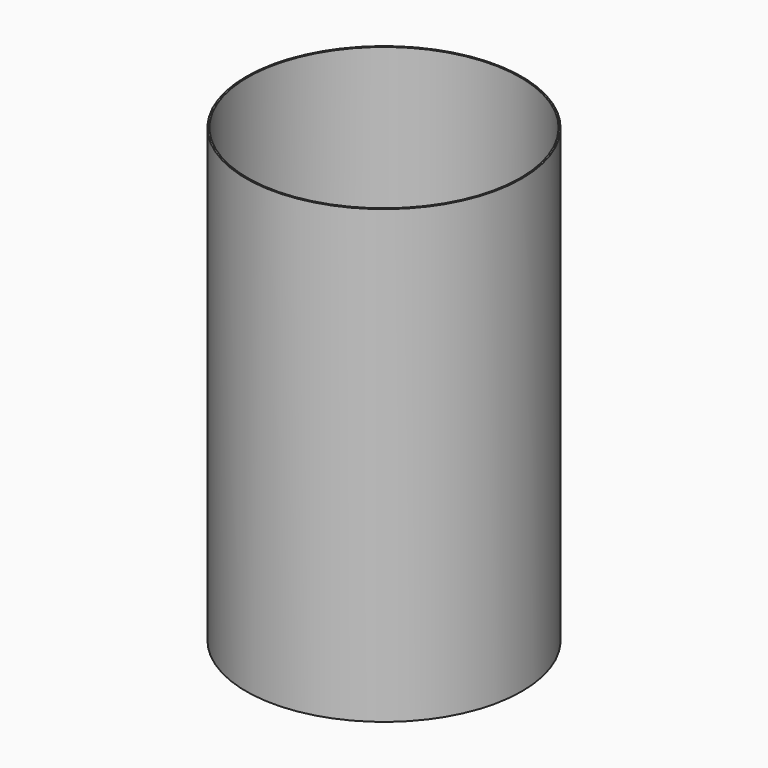
from build123d import *

# Parameters (mm, degrees)
F0_R     = 279.4
F0_R_2   = 276.225
F2_DEPTH = 914.4


# Not quite as in the source:
# - the program builds the solid bodies; features that only make, move or delete a surface that nothing else refers to are left out


with BuildPart() as f2:
    # F0 (on Top) → F2 (new body)
    with BuildSketch(Plane.XY):
        Circle(F0_R)
        Circle(F0_R_2, mode=Mode.SUBTRACT)
    extrude(amount=F2_DEPTH)


solid = f2.part
